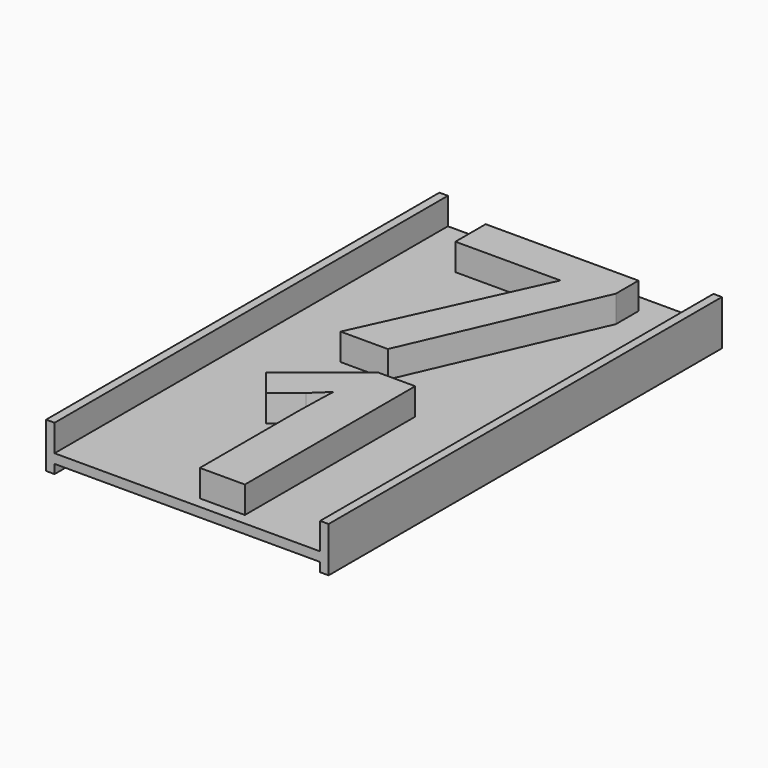
from build123d import *

# Parameters (mm, degrees)
F0_W         = 100
F0_H         = 177
F1_DEPTH     = 16
F2_W         = 94
F2_H         = 200
F3_DEPTH     = 9.5
F4_W         = 94
F4_H         = 28
F5_DEPTH     = 3.2
F6_TEXT_SIZE = 105.5555555556
F7_DEPTH     = 9.5
F9_DEPTH     = 3


# Not quite as in the source:
# - Text() gives the source's letters only with a copy of the font that has no kerning and outlines rounded to 1/6400 em; it was checked with that copy


with BuildPart() as f1:
    # F0 (on Top) → F1 (new body)
    with BuildSketch(Plane.XY):
        with Locations((50, 88.5)):
            Rectangle(F0_W, F0_H)
    extrude(amount=F1_DEPTH)

    # F2 (on face) → F3 (cut)
    with BuildSketch(Plane.XY.offset(16)):
        with Locations((50, 74)):
            Rectangle(F2_W, F2_H)
    extrude(amount=-F3_DEPTH, mode=Mode.SUBTRACT)

    # F4 (on face) → F5 (cut)
    with BuildSketch(Plane(origin=(0, 0, 0), x_dir=(1, 0, 0), z_dir=(0, 0, -1))):
        with Locations((50, -11)):
            Rectangle(F4_W, F4_H)
        with Locations((50, -163)):
            Rectangle(F4_W, F4_H)
    extrude(amount=-F5_DEPTH, mode=Mode.SUBTRACT)

    # F6 (on face) → F7 (join)
    with BuildSketch(Plane.XY.offset(6.5)):
        with Locations((18.9543402778, 92)):
            Text('7', F6_TEXT_SIZE, font='Open Sans', font_style=FontStyle.BOLD, text_align=(TextAlign.LEFT, TextAlign.BOTTOM))
        with Locations((23.5477430556, 4)):
            Text('1', F6_TEXT_SIZE, font='Open Sans', font_style=FontStyle.BOLD, text_align=(TextAlign.LEFT, TextAlign.BOTTOM))
    extrude(amount=F7_DEPTH)

    # F8 (on face) → F9 (cut)
    with BuildSketch(Plane(origin=(0, 177, 0), x_dir=(-1, 0, 0), z_dir=(0, 1, 0))):
        Polygon((-3, 0), (0, 0), (0, 16), (-100, 16), (-100, 0), (-97, 0), (-97, 3.2), (-3, 3.2), align=None)
    extrude(amount=-F9_DEPTH, mode=Mode.SUBTRACT)


solid = f1.part
